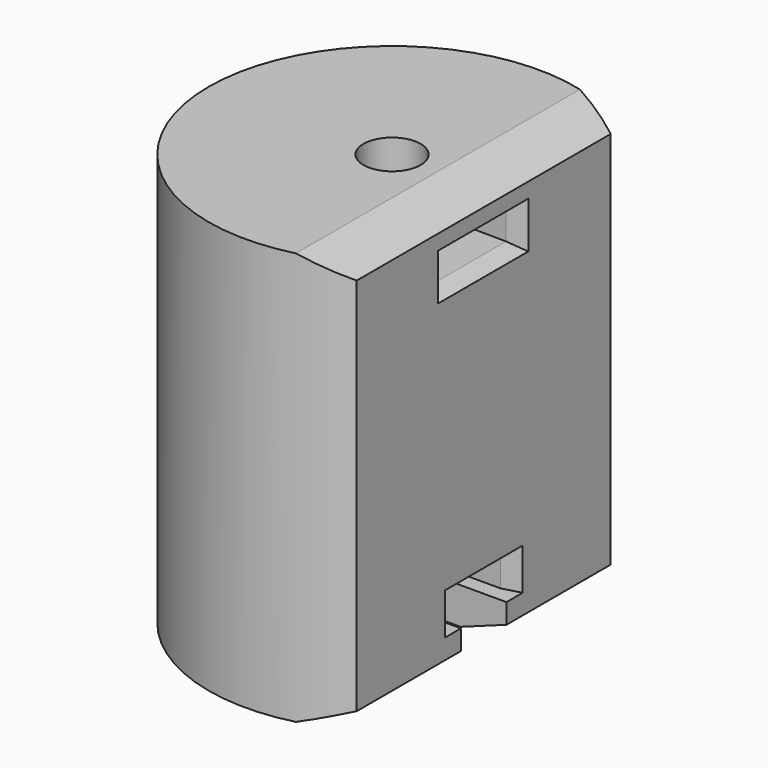
from build123d import *

# Parameters (mm, degrees)
F0_R          = 20
F1_DEPTH      = 22.5
F2_R          = 3.125
F3_DEPTH      = 4
F5_DEPTH      = 45.001
F9_DEPTH      = 4
F12_W         = 6.2
F12_H         = 4
F13_DEPTH     = 10
F14_SIZE2     = 5
F14_SIZE      = 1.8198511713
F15_T1_DEPTH  = 9.5262794416
F15_T3_DEPTH  = 4
F15_T5_DEPTH  = 4
F15_T10_DEPTH = 21.6375603763
F15_T16_DEPTH = 21.6375603763
F15_T23_DEPTH = 14.719722582
F15_T27_DEPTH = 9.1934431404
F15_T34_DEPTH = 9.1934431404
F15_T38_DEPTH = 14.719722582
F15_T45_DEPTH = 21.6375603763
F15_T49_DEPTH = 9.179576725
F15_T56_DEPTH = 21.6375603763
F15_T60_DEPTH = 9.2078904559
F15_T67_DEPTH = 9.2078904559
F15_T72_DEPTH = 21.6375603763
F15_T79_DEPTH = 9.179576725
F15_T84_DEPTH = 21.6375603763


# Not quite as in the source:
# - a fillet or chamfer that OpenCascade refuses, or shapes differently, is made with other operations: its cross-section is extruded or revolved along the edge and cut away or added


with BuildPart() as f1:
    # F0 (on Top) → F1 (new body, symmetric)
    with BuildSketch(Plane.XY):
        Circle(F0_R)
    extrude(amount=F1_DEPTH, both=True)


with BuildPart() as f3:
    # F2 (on face) → F3 (new body)
    with BuildSketch(Plane.XY.offset(22.5)):
        Polygon((4.8403136616, -2.8656567585), (4.9018883821, 2.759006214), (0.0615747205, 5.6246629725), (-4.8403136616, 2.8656567585), (-4.9018883821, -2.759006214), (-0.0615747205, -5.6246629725), align=None)
        Circle(F2_R, mode=Mode.SUBTRACT)
        Polygon((0.0615747205, 5.6246629725), (4.9018883821, 2.759006214), (4.8403136616, -2.8656567585), (-0.0615747205, -5.6246629725), (10, -5.7348097768), (10, 5.5158643187), align=None)
        Circle(F2_R)
    extrude(amount=F3_DEPTH)


with BuildPart() as f3b:
    # F2 (on face) → F3, piece 2 (new body)
    with BuildSketch(Plane.XY.offset(22.5)):
        with BuildLine():
            Line((49.1066566767, 5.0877530758), (19.2531154371, 5.4145679388))
            ThreePointArc((19.2531154371, 5.4145679388), (19.812399006, 2.7329188844), (20, 0))
            ThreePointArc((20, 0), (19.7812957099, -2.9496338823), (19.1299659961, -5.8347580061))
            Line((19.1299659961, -5.8347580061), (49.1066566767, -6.1629210197))
            Line((49.1066566767, -6.1629210197), (49.1066566767, 5.0877530758))
        make_face()
    extrude(amount=F3_DEPTH)


with BuildPart() as f3_1:
    # F4: moved
    add(f3.part.moved(Location((0, 0, -8))))


with BuildPart() as f5_tool:
    # F2 (on face) → F5 (new body, through all)
    with BuildSketch(Plane.XY.offset(22.5)):
        Circle(F2_R)
        with BuildLine():
            Line((10, 17.3205080757), (10, 5.5158643187))
            Line((10, 5.5158643187), (19.2531154371, 5.4145679388))
            ThreePointArc((19.2531154371, 5.4145679388), (15.7915814069, 12.2729766833), (10, 17.3205080757))
        make_face()
        with BuildLine():
            Line((19.2531154371, 5.4145679388), (10, 5.5158643187))
            Line((10, 5.5158643187), (10, -5.7348097768))
            Line((10, -5.7348097768), (19.1299659961, -5.8347580061))
            ThreePointArc((19.1299659961, -5.8347580061), (19.7812957099, -2.9496338823), (20, 0))
            ThreePointArc((20, 0), (19.812399006, 2.7329188844), (19.2531154371, 5.4145679388))
        make_face()
        with BuildLine():
            Line((19.1299659961, -5.8347580061), (10, -5.7348097768))
            Line((10, -5.7348097768), (10, -17.3205080757))
            ThreePointArc((10, -17.3205080757), (15.6562876634, -12.4451057288), (19.1299659961, -5.8347580061))
        make_face()
    extrude(amount=-F5_DEPTH)


with BuildPart() as f1_1:
    add(f1.part)

    # F5: cut by f5_tool
    add(f5_tool.part, mode=Mode.SUBTRACT)


with BuildPart() as f3_2:
    add(f3_1.part)

    # F5: cut by f5_tool
    add(f5_tool.part, mode=Mode.SUBTRACT)


with BuildPart() as f1_2:
    add(f1_1.part)

    # F7: cut F3
    add(f3_2.part, mode=Mode.SUBTRACT)


with BuildPart() as f9:
    # F8 (on face) → F9 (new body)
    with BuildSketch(Plane(origin=(0, 0, -22.5), x_dir=(1, 0, 0), z_dir=(0, 0, -1))):
        Polygon((22.1706703305, 4.7631397208), (10, 4.7631397208), (10, -4.7631397208), (22.864067927, -4.7631397208), align=None)
        Polygon((2.75, 4.7631397208), (5.5, 0), (3, -4.3301270189), (3, -4.7631397208), (10, -4.7631397208), (10, 4.7631397208), align=None)
        with BuildLine():
            Line((3, -4.3301270189), (5.5, 0))
            Line((5.5, 0), (2.75, 4.7631397208))
            Line((2.75, 4.7631397208), (-2.75, 4.7631397208))
            Line((-2.75, 4.7631397208), (-5.5, 0))
            Line((-5.5, 0), (-3, -4.3301270189))
            Line((-3, -4.3301270189), (-3, -0.875))
            ThreePointArc((-3, -0.875), (-0.4419417382, 3.0935921677), (3.125, 0))
            ThreePointArc((3.125, 0), (3.0935921677, -0.4419417382), (3, -0.875))
            Line((3, -0.875), (3, -4.3301270189))
        make_face()
        with BuildLine():
            Line((2.75, -4.7631397208), (3, -4.3301270189))
            Line((3, -4.3301270189), (3, -0.875))
            ThreePointArc((3, -0.875), (0, -3.125), (-3, -0.875))
            Line((-3, -0.875), (-3, -4.3301270189))
            Line((-3, -4.3301270189), (-2.75, -4.7631397208))
            Line((-2.75, -4.7631397208), (2.75, -4.7631397208))
        make_face()
    extrude(amount=F9_DEPTH)


with BuildPart() as f9_1:
    # F10: moved
    add(f9.part.moved(Location((0, 0, 8))))


with BuildPart() as f1_3:
    add(f1_2.part)

    # F11: cut F9
    add(f9_1.part, mode=Mode.SUBTRACT)

    # F12 (on face) → F13 (cut)
    with BuildSketch(Plane.YZ.offset(10)):
        with Locations((0, -20.5)):
            Rectangle(F12_W, F12_H)
    extrude(amount=-F13_DEPTH, mode=Mode.SUBTRACT)

    # F14
    f14_edges = [f1_3.edges().sort_by_distance(p)[0] for p in [
        (10, -10.210254, -22.5),
        (10, 10.210254, -22.5),
        (10, 0, 22.5),
    ]]
    f14_side = f1_3.faces().sort_by_distance((10, 0.003395, 0.271955))[0]
    chamfer(f14_edges, length=F14_SIZE, length2=F14_SIZE2, reference=f14_side)

    # F15: chamfer of 2 x 0.5358983849 on 7 edges, made by hand

    # F15_s2 → F15_t1 (cut)
    with BuildSketch(Plane.XZ.offset(-4.7631397208)):
        Polygon((10, -13.9641016151), (8, -14.5), (10, -14.5), align=None)
    extrude(amount=F15_T1_DEPTH, mode=Mode.SUBTRACT)

    # F15_s4 → F15_t3 (cut)
    with BuildSketch(Plane.XY.offset(14.5)):
        Polygon((10, 6.0736893602), (7.9941337256, 5.5378230842), (10, 5.5158643187), align=None)
        Polygon((10, -6.2488457266), (8.0058662744, -5.7129794507), (10, -5.7348097768), align=None)
    extrude(amount=F15_T3_DEPTH, mode=Mode.SUBTRACT)

    # F15_s6 → F15_t5 (cut)
    with BuildSketch(Plane.XY.offset(-18.5)):
        Polygon((10, -5.2990381057), (8, -4.7631397208), (10, -4.7631397208), align=None)
        Polygon((10, 5.2990381057), (8, 4.7631397208), (10, 4.7631397208), align=None)
    extrude(amount=F15_T5_DEPTH, mode=Mode.SUBTRACT)


with BuildPart() as f15_tool8:
    # F15_s9 → F15_t10 (new body)
    with BuildSketch(Plane.XZ.offset(10.9282529172)):
        Polygon((10, 13.9641016151), (8, 14.5), (10, 14.5), align=None)
    extrude(amount=-F15_T10_DEPTH)

    split(bisect_by=Plane(origin=(-0.0615747205, -5.6246629725, 0), x_dir=(0, 0, 1), z_dir=(0.010946617, 0.999940084, 0)), keep=Keep.TOP)

    split(bisect_by=Plane(origin=(0.0615747205, 5.6246629725, 0), x_dir=(0, 0, 1), z_dir=(-0.010946617, -0.999940084, 0)), keep=Keep.TOP)


with BuildPart() as f1_4:
    add(f1_3.part)

    # F15_t7: cut F15_tool8
    add(f15_tool8.part, mode=Mode.SUBTRACT)


with BuildPart() as f15_tool14:
    # F15_s15 → F15_t16 (new body)
    with BuildSketch(Plane.XZ.offset(10.9282529172)):
        Polygon((10, 19.0358983849), (8, 18.5), (10, 18.5), align=None)
    extrude(amount=-F15_T16_DEPTH)

    split(bisect_by=Plane(origin=(-0.0615747205, -5.6246629725, 0), x_dir=(0, 0, 1), z_dir=(0.010946617, 0.999940084, 0)), keep=Keep.TOP)

    split(bisect_by=Plane(origin=(0.0615747205, 5.6246629725, 0), x_dir=(0, 0, 1), z_dir=(-0.010946617, -0.999940084, 0)), keep=Keep.TOP)


with BuildPart() as f1_5:
    add(f1_4.part)

    # F15_t13: cut F15_tool14
    add(f15_tool14.part, mode=Mode.SUBTRACT)


with BuildPart() as f15_tool21:
    # F15_s22 → F15_t23 (new body)
    with BuildSketch(Plane.XZ.offset(-9.9565828612)):
        Polygon((10, -13.9641016151), (8, -14.5), (10, -14.5), align=None)
    extrude(amount=F15_T23_DEPTH)

    split(bisect_by=Plane.XZ.offset(-4.7631397208), keep=Keep.BOTTOM)


with BuildPart() as f15_tool25:
    # F15_s26 → F15_t27 (new body)
    with BuildSketch(Plane.XY.offset(-18.5)):
        Polygon((10, 5.2990381057), (8, 4.7631397208), (10, 4.7631397208), align=None)
    extrude(amount=F15_T27_DEPTH)

    split(bisect_by=Plane.XY.offset(-14.5), keep=Keep.TOP)


with BuildPart() as f15_tool21_1:
    add(f15_tool21.part)

    # F15_t29: intersect F15_tool25
    add(f15_tool25.part, mode=Mode.INTERSECT)


with BuildPart() as f1_6:
    add(f1_5.part)

    # F15_t19: cut F15_tool21
    add(f15_tool21_1.part, mode=Mode.SUBTRACT)


with BuildPart() as f15_tool32:
    # F15_s33 → F15_t34 (new body)
    with BuildSketch(Plane.XY.offset(-9.3065568596)):
        Polygon((10, -5.2990381057), (8, -4.7631397208), (10, -4.7631397208), align=None)
    extrude(amount=-F15_T34_DEPTH)

    split(bisect_by=Plane.XY.offset(-14.5), keep=Keep.TOP)


with BuildPart() as f15_tool36:
    # F15_s37 → F15_t38 (new body)
    with BuildSketch(Plane.XZ.offset(-4.7631397208)):
        Polygon((10, -13.9641016151), (8, -14.5), (10, -14.5), align=None)
    extrude(amount=F15_T38_DEPTH)

    split(bisect_by=Plane.XZ.offset(4.7631397208), keep=Keep.TOP)


with BuildPart() as f15_tool32_1:
    add(f15_tool32.part)

    # F15_t40: intersect F15_tool36
    add(f15_tool36.part, mode=Mode.INTERSECT)


with BuildPart() as f1_7:
    add(f1_6.part)

    # F15_t30: cut F15_tool32
    add(f15_tool32_1.part, mode=Mode.SUBTRACT)


with BuildPart() as f15_tool43:
    # F15_s44 → F15_t45 (new body)
    with BuildSketch(Plane.XZ.offset(10.9282529172)):
        Polygon((10, 13.9641016151), (8, 14.5), (10, 14.5), align=None)
    extrude(amount=-F15_T45_DEPTH)

    split(bisect_by=Plane(origin=(-0.0615747205, -5.6246629725, 0), x_dir=(0, 0, 1), z_dir=(-0.010946617, -0.999940084, 0)), keep=Keep.TOP)


with BuildPart() as f15_tool47:
    # F15_s48 → F15_t49 (new body)
    with BuildSketch(Plane.XY.offset(9.320423275)):
        Polygon((10, -6.2488457266), (8.0058662744, -5.7129794507), (10, -5.7348097768), align=None)
    extrude(amount=F15_T49_DEPTH)

    split(bisect_by=Plane.XY.offset(14.5), keep=Keep.BOTTOM)


with BuildPart() as f15_tool43_1:
    add(f15_tool43.part)

    # F15_t51: intersect F15_tool47
    add(f15_tool47.part, mode=Mode.INTERSECT)


with BuildPart() as f1_8:
    add(f1_7.part)

    # F15_t41: cut F15_tool43
    add(f15_tool43_1.part, mode=Mode.SUBTRACT)


with BuildPart() as f15_tool54:
    # F15_s55 → F15_t56 (new body)
    with BuildSketch(Plane.XZ.offset(10.9282529172)):
        Polygon((10, 13.9641016151), (8, 14.5), (10, 14.5), align=None)
    extrude(amount=-F15_T56_DEPTH)

    split(bisect_by=Plane(origin=(0.0615747205, 5.6246629725, 0), x_dir=(0, 0, 1), z_dir=(0.010946617, 0.999940084, 0)), keep=Keep.TOP)


with BuildPart() as f15_tool58:
    # F15_s59 → F15_t60 (new body)
    with BuildSketch(Plane.XY.offset(9.2921095441)):
        Polygon((10, 6.0736893602), (7.9941337256, 5.5378230842), (10, 5.5158643187), align=None)
    extrude(amount=F15_T60_DEPTH)

    split(bisect_by=Plane.XY.offset(14.5), keep=Keep.BOTTOM)


with BuildPart() as f15_tool54_1:
    add(f15_tool54.part)

    # F15_t62: intersect F15_tool58
    add(f15_tool58.part, mode=Mode.INTERSECT)


with BuildPart() as f1_9:
    add(f1_8.part)

    # F15_t52: cut F15_tool54
    add(f15_tool54_1.part, mode=Mode.SUBTRACT)


with BuildPart() as f15_tool65:
    # F15_s66 → F15_t67 (new body)
    with BuildSketch(Plane.XY.offset(14.5)):
        Polygon((10, 6.0736893602), (7.9941337256, 5.5378230842), (10, 5.5158643187), align=None)
    extrude(amount=F15_T67_DEPTH)

    split(bisect_by=Plane(origin=(7.8162495012, 0, 21.4749690093), x_dir=(0, 1, 0), z_dir=(-0.3420201433, 0, -0.9396926208)), keep=Keep.TOP)

    split(bisect_by=Plane.XY.offset(18.5), keep=Keep.TOP)


with BuildPart() as f15_tool70:
    # F15_s71 → F15_t72 (new body)
    with BuildSketch(Plane.XZ.offset(10.9282529172)):
        Polygon((10, 19.0358983849), (8, 18.5), (10, 18.5), align=None)
    extrude(amount=-F15_T72_DEPTH)

    split(bisect_by=Plane(origin=(0.0615747205, 5.6246629725, 0), x_dir=(0, 0, 1), z_dir=(0.010946617, 0.999940084, 0)), keep=Keep.TOP)


with BuildPart() as f15_tool65_1:
    add(f15_tool65.part)

    # F15_t74: intersect F15_tool70
    add(f15_tool70.part, mode=Mode.INTERSECT)


with BuildPart() as f1_10:
    add(f1_9.part)

    # F15_t63: cut F15_tool65
    add(f15_tool65_1.part, mode=Mode.SUBTRACT)


with BuildPart() as f15_tool77:
    # F15_s78 → F15_t79 (new body)
    with BuildSketch(Plane.XY.offset(14.5)):
        Polygon((10, -6.2488457266), (8.0058662744, -5.7129794507), (10, -5.7348097768), align=None)
    extrude(amount=F15_T79_DEPTH)

    split(bisect_by=Plane(origin=(7.8162495012, 0, 21.4749690093), x_dir=(0, 1, 0), z_dir=(-0.3420201433, 0, -0.9396926208)), keep=Keep.TOP)

    split(bisect_by=Plane.XY.offset(18.5), keep=Keep.TOP)


with BuildPart() as f15_tool82:
    # F15_s83 → F15_t84 (new body)
    with BuildSketch(Plane.XZ.offset(10.9282529172)):
        Polygon((10, 19.0358983849), (8, 18.5), (10, 18.5), align=None)
    extrude(amount=-F15_T84_DEPTH)

    split(bisect_by=Plane(origin=(-0.0615747205, -5.6246629725, 0), x_dir=(0, 0, 1), z_dir=(-0.010946617, -0.999940084, 0)), keep=Keep.TOP)


with BuildPart() as f15_tool77_1:
    add(f15_tool77.part)

    # F15_t86: intersect F15_tool82
    add(f15_tool82.part, mode=Mode.INTERSECT)


with BuildPart() as f1_11:
    add(f1_10.part)

    # F15_t75: cut F15_tool77
    add(f15_tool77_1.part, mode=Mode.SUBTRACT)


solid = f1_11.part
